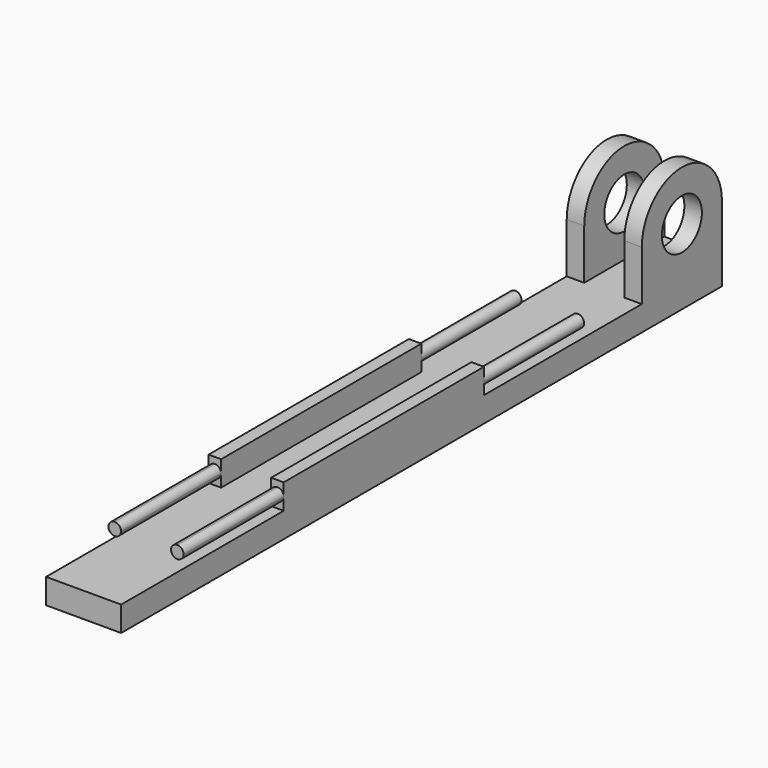
from build123d import *

# Parameters (mm, degrees)
F0_W      = 6
F0_H      = 60
F1_DEPTH  = 2
F3_DEPTH  = 6
F6_DEPTH  = 25
F4_W      = 1
F4_H      = 20
F7_DEPTH  = 2
F9_DEPTH  = 10
F10_R     = 0.5
F11_DEPTH = 10


# Not quite as in the source:
# - a feature of the source that left no trace in its solid (it failed there, or was rolled back) is left out
# - the program builds the solid bodies; features that only make, move or delete a surface that nothing else refers to are left out


with BuildPart() as f1:
    # F0 (on Top) → F1 (new body)
    with BuildSketch(Plane.XY):
        Rectangle(F0_W, F0_H)
    extrude(amount=F1_DEPTH)

    # F2 (on face) → F3 (join)
    with BuildSketch(Plane.YZ.offset(3)):
        with BuildLine():
            Line((28, 6), (30, 6))
            ThreePointArc((30, 6), (26, 10), (22, 6))
            Line((22, 6), (24, 6))
            ThreePointArc((24, 6), (26, 8), (28, 6))
        make_face()
        with BuildLine():
            Line((22, 2), (30, 2))
            Line((30, 2), (30, 6))
            Line((30, 6), (28, 6))
            ThreePointArc((28, 6), (26, 4), (24, 6))
            Line((24, 6), (22, 6))
            Line((22, 6), (22, 2))
        make_face()
    extrude(amount=-F3_DEPTH)

    # F5 (on face) → F6 (cut)
    with BuildSketch(Plane.XY.offset(2)):
        Polygon((1.6, 22), (1.6, 30), (0, 30), (-1.6, 30), (-1.6, 22), align=None)
    extrude(amount=F6_DEPTH, mode=Mode.SUBTRACT)

    # F4 (on face) → F7 (join)
    with BuildSketch(Plane.XY.offset(2)):
        with Locations((2.5, -3.7680014595)):
            Rectangle(F4_W, F4_H)
        with Locations((-2.5, -3.7680014595)):
            Rectangle(F4_W, F4_H)
    extrude(amount=F7_DEPTH)

    # F8 (on face) → F9 (join)
    with BuildSketch(Plane.XZ.offset(13.7680014595)):
        with BuildLine():
            ThreePointArc((2.5, 3.5), (2.1464466094, 3.3535533906), (2, 3))
            ThreePointArc((2, 3), (2.5, 2.5), (3, 3))
            ThreePointArc((3, 3), (2.8535533906, 3.3535533906), (2.5, 3.5))
        make_face()
        with BuildLine():
            ThreePointArc((-2.5, 3.5), (-2.8535533906, 2.6464466094), (-2, 3))
            ThreePointArc((-2, 3), (-2.1464466094, 3.3535533906), (-2.5, 3.5))
        make_face()
    extrude(amount=F9_DEPTH)

    # F10 (on face) → F11 (join)
    with BuildSketch(Plane(origin=(0, 6.2319985405, 0), x_dir=(-1, 0, 0), z_dir=(0, 1, 0))):
        with Locations((-2.5, 3)):
            Circle(F10_R)
        with Locations((2.5, 3)):
            Circle(F10_R)
    extrude(amount=F11_DEPTH)


solid = f1.part
